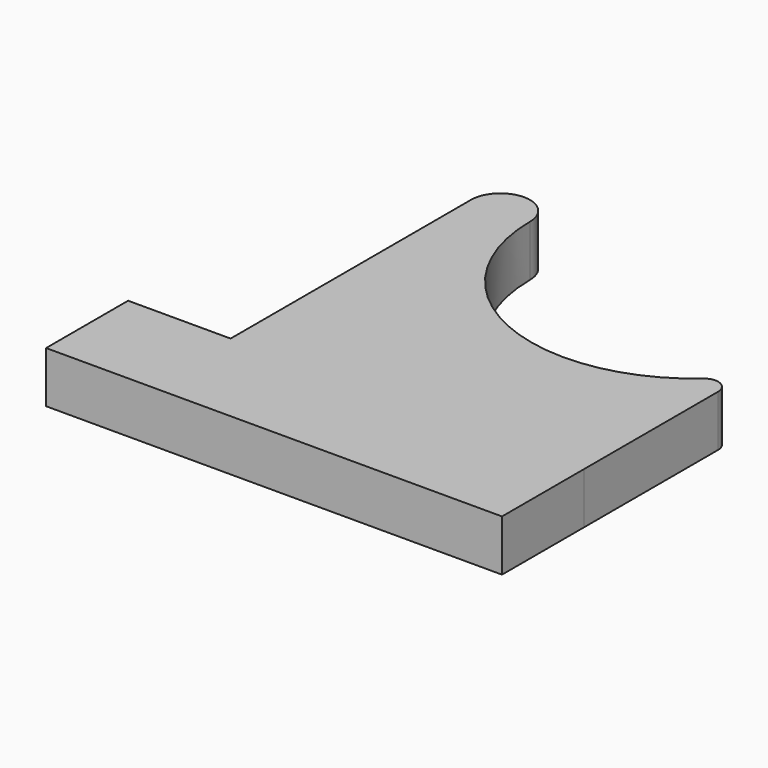
from build123d import *

# Parameters (mm, degrees)
F1_DEPTH = 5
F2_W     = 34.4714387385
F2_H     = 10
F2_W_2   = 10
F3_DEPTH = 5


# Not quite as in the source:
# - ends of sketch curves that miss each other by under 0.0002 mm in the source are joined


with BuildPart() as f1:
    # F0 (on Top) → F1 (new body)
    with BuildSketch(Plane.XY):
        with BuildLine():
            Line((0, 29.2999204248), (0, 0))
            Line((0, 0), (34.4714387385, 0))
            Line((34.4714387385, 0), (34.4714387385, 16.3473710418))
            ThreePointArc((34.4714387385, 16.3473710418), (32.5790927131, 15.1300794804), (32.2559916738, 17.3568210333))
            ThreePointArc((32.2559916738, 17.3568210333), (15.182844974, 14.8438668457), (5.7578901922, 29.2999210911))
            ThreePointArc((5.7578901922, 29.2999210911), (2.8789043427, 26.4210160822), (0, 29.2999204248))
        make_face()
        with BuildLine():
            ThreePointArc((5.7577396052, 29.3198639813), (2.8689325046, 32.1788074974), (0, 29.2999204248))
            ThreePointArc((0, 29.2999204248), (2.8789043427, 26.4210160822), (5.7578086853, 29.2999204248))
            ThreePointArc((5.7578086853, 29.2999204248), (5.7578117914, 29.3098925127), (5.7577396052, 29.3198639813))
        make_face()
        with BuildLine():
            ThreePointArc((32.2559916738, 17.3568210333), (32.5790927131, 15.1300794804), (34.4714387385, 16.3473710418))
            ThreePointArc((34.4714387385, 16.3473710418), (33.6883902233, 17.5646626032), (32.2559916738, 17.3568210333))
        make_face()
    extrude(amount=F1_DEPTH)

    # F2 (on face) → F3 (join)
    with BuildSketch(Plane.XY.offset(5)):
        with BuildLine():
            Line((0, 0), (34.4714387385, 0))
            Line((34.4714387385, 0), (34.4714387385, 16.3473710418))
            ThreePointArc((34.4714387385, 16.3473710418), (33.6883902233, 17.5646626032), (32.2559916738, 17.3568210333))
            ThreePointArc((32.2559916738, 17.3568210333), (15.182844974, 14.8438668457), (5.7578901922, 29.2999210911))
            ThreePointArc((5.7578901922, 29.2999210911), (5.757811792, 29.3098923335), (5.7577396052, 29.3198639813))
            ThreePointArc((5.7577396052, 29.3198639813), (2.8689325046, 32.1788074974), (0, 29.2999204248))
            Line((0, 29.2999204248), (0, 25.4882741719))
            Line((0, 25.4882741719), (0, 0))
        make_face()
        with Locations((17.2357193692, -5)):
            Rectangle(F2_W, F2_H)
        with Locations((-5, -5)):
            Rectangle(F2_W_2, F2_H)
        with Locations((-5, -5)):
            Rectangle(F2_W_2, F2_H)
    extrude(amount=-F3_DEPTH)


solid = f1.part
